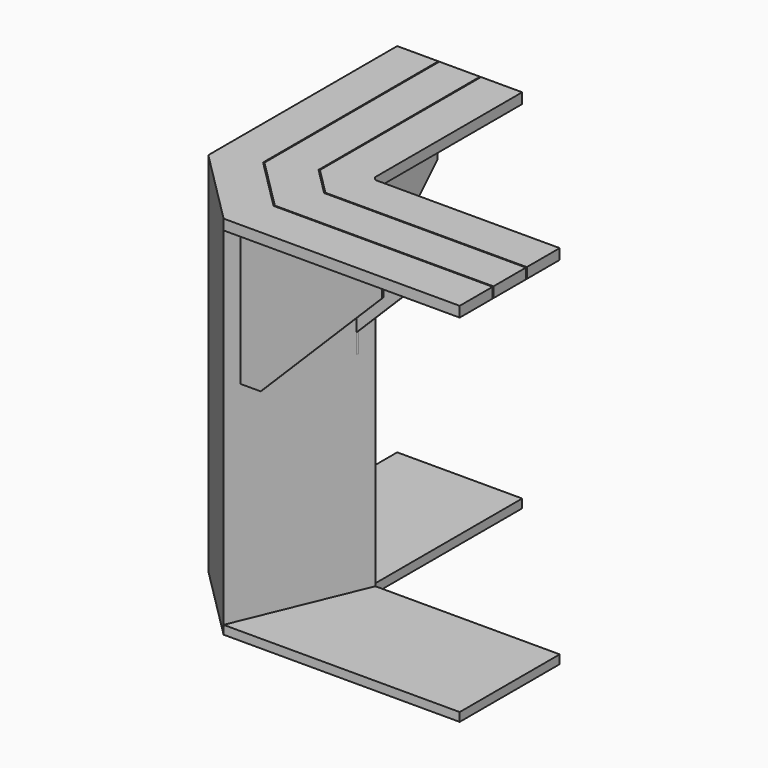
from build123d import *

# Parameters (mm, degrees)
F1_DEPTH     = 30
F3_DEPTH     = 1000
F5_DEPTH     = 25
F6_W         = 5
F6_H         = 408.0812203564
F7_DEPTH     = 400
F8_T4_DEPTH  = 1805.1780915761
F8_T10_DEPTH = 1805.1780915761
F8_T16_DEPTH = 1805.1780915761
F8_T22_DEPTH = 1805.1780915761
F8_T28_DEPTH = 1805.1780915761
F8_T34_DEPTH = 1805.1780915761
F8_T40_DEPTH = 1805.1780915761
F8_T46_DEPTH = 1805.1780915761
F8_T52_DEPTH = 1805.1780915761
F8_T58_DEPTH = 1805.1780915761
F8_T64_DEPTH = 1805.1780915761
F8_T70_DEPTH = 1805.1780915761
F12_DEPTH    = 30
F13_DEPTH    = 5


# Not quite as in the source:
# - a fillet or chamfer that OpenCascade refuses, or shapes differently, is made with other operations: its cross-section is extruded or revolved along the edge and cut away or added


with BuildPart() as f1:
    # F0 (on Top) → F1 (new body)
    with BuildSketch(Plane.XY):
        Polygon((-190, 550), (-550, 550), (-550, -130), (-330, -350), (350, -350), (350, 10), (-180.8831175457, 10), (-190, 19.1168824543), align=None)
    extrude(amount=F1_DEPTH)

    # F2 (on face) → F3 (join)
    with BuildSketch(Plane(origin=(0, 0, 0), x_dir=(1, 0, 0), z_dir=(0, 0, -1))):
        Polygon((-330, 350), (-550, 130), (-190, -19.1168824543), (-180.8831175457, -10), align=None)
    extrude(amount=F3_DEPTH)

    # F4 (on face) → F5 (join)
    with BuildSketch(Plane(origin=(0, 0, -1000), x_dir=(1, 0, 0), z_dir=(0, 0, -1))):
        Polygon((350, 350), (-330, 350), (-550, 130), (-550, -550), (-190, -550), (-190, -19.1168824543), (-180.8831175457, -10), (350, -10), align=None)
    extrude(amount=F5_DEPTH)

    # F6 (on face) → F7 (join)
    with BuildSketch(Plane(origin=(0, 0, 0), x_dir=(1, 0, 0), z_dir=(0, 0, -1))):
        Polygon((-311.3603896932, 305), (94.6497628513, 305), (94.6497628513, 310), (-313.4314575051, 310), align=None)
        with Locations((-507.5, -90.6091526731)):
            Rectangle(F6_W, F6_H)
        Polygon((94.6497628513, 30), (94.6497628513, 35), (-199.5227278525, 35), (-197.4516600406, 30), align=None)
        Polygon((-235, -0.4772721475), (-235, -294.6497628513), (-230, -294.6497628513), (-230, -2.5483399594), align=None)
    extrude(amount=F7_DEPTH)

    # F8: chamfer of 350 on 4 edges, made by hand


with BuildPart() as f8_tool2:
    # F8_s3 → F8_t4 (new body)
    with BuildSketch(Plane.YZ.offset(-1410.0890457881)):
        Polygon((-55.3502371487, -400), (294.6497628513, -50), (294.6497628513, -400), align=None)
    extrude(amount=F8_T4_DEPTH)

    split(bisect_by=Plane(origin=(-34.5836943966, 83.4924240492, 0), x_dir=(0, 0, 1), z_dir=(-0.3826834324, 0.9238795325, 0)), keep=Keep.TOP)

    split(bisect_by=Plane(origin=(-157.9289321881, 65.4163056034, 0), x_dir=(0, 0, 1), z_dir=(-0.9238795325, 0.3826834324, 0)), keep=Keep.TOP)


with BuildPart() as f1_1:
    add(f1.part)

    # F8_t1: cut F8_tool2
    add(f8_tool2.part, mode=Mode.SUBTRACT)


with BuildPart() as f8_tool8:
    # F8_s9 → F8_t10 (new body)
    with BuildSketch(Plane.YZ.offset(-1410.0890457881)):
        Polygon((-55.3502371487, -400), (294.6497628513, -50), (294.6497628513, -400), align=None)
    extrude(amount=F8_T10_DEPTH)

    split(bisect_by=Plane(origin=(-34.5836943966, 83.4924240492, 0), x_dir=(0, 0, 1), z_dir=(-0.3826834324, 0.9238795325, 0)), keep=Keep.TOP)

    split(bisect_by=Plane(origin=(-157.9289321881, 65.4163056034, 0), x_dir=(0, 0, 1), z_dir=(0.9238795325, -0.3826834324, 0)), keep=Keep.TOP)


with BuildPart() as f1_2:
    add(f1_1.part)

    # F8_t7: cut F8_tool8
    add(f8_tool8.part, mode=Mode.SUBTRACT)


with BuildPart() as f8_tool14:
    # F8_s15 → F8_t16 (new body)
    with BuildSketch(Plane.YZ.offset(-1410.0890457881)):
        Polygon((-55.3502371487, -400), (294.6497628513, -50), (294.6497628513, -400), align=None)
    extrude(amount=F8_T16_DEPTH)

    split(bisect_by=Plane(origin=(-34.5836943966, 83.4924240492, 0), x_dir=(0, 0, 1), z_dir=(0.3826834324, -0.9238795325, 0)), keep=Keep.TOP)

    split(bisect_by=Plane(origin=(-157.9289321881, 65.4163056034, 0), x_dir=(0, 0, 1), z_dir=(0.9238795325, -0.3826834324, 0)), keep=Keep.TOP)


with BuildPart() as f1_3:
    add(f1_2.part)

    # F8_t13: cut F8_tool14
    add(f8_tool14.part, mode=Mode.SUBTRACT)


with BuildPart() as f8_tool20:
    # F8_s21 → F8_t22 (new body)
    with BuildSketch(Plane.XZ.offset(-595.0890457881)):
        Polygon((-255.3502371487, -400), (94.6497628513, -50), (94.6497628513, -400), align=None)
    extrude(amount=F8_T22_DEPTH)

    split(bisect_by=Plane(origin=(-34.5836943966, 83.4924240492, 0), x_dir=(0, 0, 1), z_dir=(-0.3826834324, 0.9238795325, 0)), keep=Keep.TOP)

    split(bisect_by=Plane(origin=(-157.9289321881, 65.4163056034, 0), x_dir=(0, 0, 1), z_dir=(-0.9238795325, 0.3826834324, 0)), keep=Keep.TOP)


with BuildPart() as f1_4:
    add(f1_3.part)

    # F8_t19: cut F8_tool20
    add(f8_tool20.part, mode=Mode.SUBTRACT)


with BuildPart() as f8_tool26:
    # F8_s27 → F8_t28 (new body)
    with BuildSketch(Plane.XZ.offset(-595.0890457881)):
        Polygon((-255.3502371487, -400), (94.6497628513, -50), (94.6497628513, -400), align=None)
    extrude(amount=F8_T28_DEPTH)

    split(bisect_by=Plane(origin=(-34.5836943966, 83.4924240492, 0), x_dir=(0, 0, 1), z_dir=(-0.3826834324, 0.9238795325, 0)), keep=Keep.TOP)

    split(bisect_by=Plane(origin=(-157.9289321881, 65.4163056034, 0), x_dir=(0, 0, 1), z_dir=(0.9238795325, -0.3826834324, 0)), keep=Keep.TOP)


with BuildPart() as f1_5:
    add(f1_4.part)

    # F8_t25: cut F8_tool26
    add(f8_tool26.part, mode=Mode.SUBTRACT)


with BuildPart() as f8_tool32:
    # F8_s33 → F8_t34 (new body)
    with BuildSketch(Plane.XZ.offset(-595.0890457881)):
        Polygon((-255.3502371487, -400), (94.6497628513, -50), (94.6497628513, -400), align=None)
    extrude(amount=F8_T34_DEPTH)

    split(bisect_by=Plane(origin=(-34.5836943966, 83.4924240492, 0), x_dir=(0, 0, 1), z_dir=(0.3826834324, -0.9238795325, 0)), keep=Keep.TOP)

    split(bisect_by=Plane(origin=(-157.9289321881, 65.4163056034, 0), x_dir=(0, 0, 1), z_dir=(0.9238795325, -0.3826834324, 0)), keep=Keep.TOP)


with BuildPart() as f1_6:
    add(f1_5.part)

    # F8_t31: cut F8_tool32
    add(f8_tool32.part, mode=Mode.SUBTRACT)


with BuildPart() as f8_tool38:
    # F8_s39 → F8_t40 (new body)
    with BuildSketch(Plane.YZ.offset(-1135.0890457881)):
        Polygon((-55.3502371487, -400), (294.6497628513, -50), (294.6497628513, -400), align=None)
    extrude(amount=F8_T40_DEPTH)

    split(bisect_by=Plane(origin=(-34.5836943966, 83.4924240492, 0), x_dir=(0, 0, 1), z_dir=(-0.3826834324, 0.9238795325, 0)), keep=Keep.TOP)

    split(bisect_by=Plane(origin=(-157.9289321881, 65.4163056034, 0), x_dir=(0, 0, 1), z_dir=(-0.9238795325, 0.3826834324, 0)), keep=Keep.TOP)


with BuildPart() as f1_7:
    add(f1_6.part)

    # F8_t37: cut F8_tool38
    add(f8_tool38.part, mode=Mode.SUBTRACT)


with BuildPart() as f8_tool44:
    # F8_s45 → F8_t46 (new body)
    with BuildSketch(Plane.YZ.offset(-1135.0890457881)):
        Polygon((-55.3502371487, -400), (294.6497628513, -50), (294.6497628513, -400), align=None)
    extrude(amount=F8_T46_DEPTH)

    split(bisect_by=Plane(origin=(-34.5836943966, 83.4924240492, 0), x_dir=(0, 0, 1), z_dir=(-0.3826834324, 0.9238795325, 0)), keep=Keep.TOP)

    split(bisect_by=Plane(origin=(-157.9289321881, 65.4163056034, 0), x_dir=(0, 0, 1), z_dir=(0.9238795325, -0.3826834324, 0)), keep=Keep.TOP)


with BuildPart() as f1_8:
    add(f1_7.part)

    # F8_t43: cut F8_tool44
    add(f8_tool44.part, mode=Mode.SUBTRACT)


with BuildPart() as f8_tool50:
    # F8_s51 → F8_t52 (new body)
    with BuildSketch(Plane.YZ.offset(-1135.0890457881)):
        Polygon((-55.3502371487, -400), (294.6497628513, -50), (294.6497628513, -400), align=None)
    extrude(amount=F8_T52_DEPTH)

    split(bisect_by=Plane(origin=(-34.5836943966, 83.4924240492, 0), x_dir=(0, 0, 1), z_dir=(0.3826834324, -0.9238795325, 0)), keep=Keep.TOP)

    split(bisect_by=Plane(origin=(-157.9289321881, 65.4163056034, 0), x_dir=(0, 0, 1), z_dir=(0.9238795325, -0.3826834324, 0)), keep=Keep.TOP)


with BuildPart() as f1_9:
    add(f1_8.part)

    # F8_t49: cut F8_tool50
    add(f8_tool50.part, mode=Mode.SUBTRACT)


with BuildPart() as f8_tool56:
    # F8_s57 → F8_t58 (new body)
    with BuildSketch(Plane.XZ.offset(-870.0890457881)):
        Polygon((-255.3502371487, -400), (94.6497628513, -50), (94.6497628513, -400), align=None)
    extrude(amount=F8_T58_DEPTH)

    split(bisect_by=Plane(origin=(-34.5836943966, 83.4924240492, 0), x_dir=(0, 0, 1), z_dir=(-0.3826834324, 0.9238795325, 0)), keep=Keep.TOP)

    split(bisect_by=Plane(origin=(-157.9289321881, 65.4163056034, 0), x_dir=(0, 0, 1), z_dir=(-0.9238795325, 0.3826834324, 0)), keep=Keep.TOP)


with BuildPart() as f1_10:
    add(f1_9.part)

    # F8_t55: cut F8_tool56
    add(f8_tool56.part, mode=Mode.SUBTRACT)


with BuildPart() as f8_tool62:
    # F8_s63 → F8_t64 (new body)
    with BuildSketch(Plane.XZ.offset(-870.0890457881)):
        Polygon((-255.3502371487, -400), (94.6497628513, -50), (94.6497628513, -400), align=None)
    extrude(amount=F8_T64_DEPTH)

    split(bisect_by=Plane(origin=(-34.5836943966, 83.4924240492, 0), x_dir=(0, 0, 1), z_dir=(-0.3826834324, 0.9238795325, 0)), keep=Keep.TOP)

    split(bisect_by=Plane(origin=(-157.9289321881, 65.4163056034, 0), x_dir=(0, 0, 1), z_dir=(0.9238795325, -0.3826834324, 0)), keep=Keep.TOP)


with BuildPart() as f1_11:
    add(f1_10.part)

    # F8_t61: cut F8_tool62
    add(f8_tool62.part, mode=Mode.SUBTRACT)


with BuildPart() as f8_tool68:
    # F8_s69 → F8_t70 (new body)
    with BuildSketch(Plane.XZ.offset(-870.0890457881)):
        Polygon((-255.3502371487, -400), (94.6497628513, -50), (94.6497628513, -400), align=None)
    extrude(amount=F8_T70_DEPTH)

    split(bisect_by=Plane(origin=(-34.5836943966, 83.4924240492, 0), x_dir=(0, 0, 1), z_dir=(0.3826834324, -0.9238795325, 0)), keep=Keep.TOP)

    split(bisect_by=Plane(origin=(-157.9289321881, 65.4163056034, 0), x_dir=(0, 0, 1), z_dir=(0.9238795325, -0.3826834324, 0)), keep=Keep.TOP)


with BuildPart() as f1_12:
    add(f1_11.part)

    # F8_t67: cut F8_tool68
    add(f8_tool68.part, mode=Mode.SUBTRACT)

    # F11 (on face) → F12 (cut, through all)
    with BuildSketch(Plane.XY.offset(30)):
        Polygon((-431.5, -80.9156928588), (-280.9156928588, -231.5), (350, -231.5), (350, -228.5), (-279.6730521717, -228.5), (-428.5, -79.6730521717), (-428.5, 550), (-431.5, 550), align=None)
        Polygon((-311.5, -31.210065374), (-231.210065374, -111.5), (350, -111.5), (350, -108.5), (-229.9674246869, -108.5), (-308.5, -29.9674246869), (-308.5, 550), (-311.5, 550), align=None)
    extrude(amount=-F12_DEPTH, mode=Mode.SUBTRACT)

    # F9 (on face) → F13 (join)
    with BuildSketch(Plane(origin=(0, 0, 0), x_dir=(1, 0, 0), z_dir=(0, 0, -1))):
        Polygon((94.6497628513, 255), (94.6497628513, 305), (-311.3603896932, 305), (-290.6497115746, 255), (44.6497628513, 255), (44.6497628513, 85), (-220.2334059711, 85), (-199.5227278525, 35), (94.6497628513, 35), (94.6497628513, 85), align=None)
        Polygon((-285, -294.6497628513), (-235, -294.6497628513), (-235, -0.4772721475), (-285, 20.2334059711), (-285, -244.6497628513), (-455, -244.6497628513), (-455, 90.6497115746), (-505, 111.3603896932), (-505, -294.6497628513), (-455, -294.6497628513), align=None)
    extrude(amount=F13_DEPTH)


solid = f1_12.part
